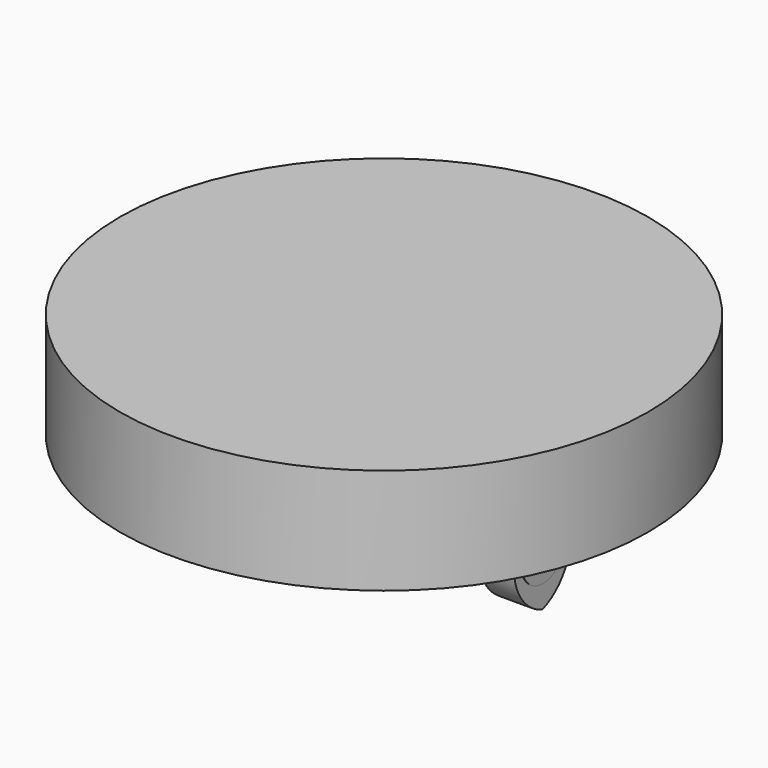
from build123d import *

# Parameters (mm, degrees)
F0_R        = 3.7479112611
F1_DEPTH    = 1.5
F3_DEPTH    = 1.5
F5_D        = 0.75
F6_T1_DEPTH = 4.2451243754
F8_R        = 0.375
F9_DEPTH    = 4.5


# Not quite as in the source:
# - a fillet or chamfer that OpenCascade refuses, or shapes differently, is made with other operations: its cross-section is extruded or revolved along the edge and cut away or added


with BuildPart() as f1:
    # F0 (on Top) → F1 (new body)
    with BuildSketch(Plane.XY):
        Circle(F0_R)
    extrude(amount=-F1_DEPTH)

    # F2 (on face) → F3 (join)
    with BuildSketch(Plane(origin=(0, 0, -1.5), x_dir=(1, 0, 0), z_dir=(0, 0, -1))):
        Polygon((-2.2448661039, -0.5004639388), (-1.7497417284, -0.5004639388), (-1.7497417284, 0), (-1.7497417284, 0.5004639388), (-2.2448661039, 0.5004639388), align=None)
    extrude(amount=F3_DEPTH)

    # F5 (through all)
    with Locations(Plane.YZ.offset(-1.7497417284)):
        with Locations((0, -2.2526816465)):
            Hole(F5_D / 2)

    # F6: fillet of radius 0.75 on 2 edges, made by hand

    # F6_s2 → F6_t1 (cut)
    with BuildSketch(Plane.YZ.offset(-4.1198661039)):
        with BuildLine():
            ThreePointArc((-0.5004639388, -2.25), (-0.2807940247, -2.7803300859), (0.2495360612, -3))
            Line((0.2495360612, -3), (-0.5004639388, -3))
            Line((-0.5004639388, -3), (-0.5004639388, -2.25))
        make_face()
        with BuildLine():
            ThreePointArc((0.5004639388, -2.25), (0.2807940247, -2.7803300859), (-0.2495360612, -3))
            Line((-0.2495360612, -3), (0.5004639388, -3))
            Line((0.5004639388, -3), (0.5004639388, -2.25))
        make_face()
    extrude(amount=F6_T1_DEPTH, mode=Mode.SUBTRACT)

    # F7: F1 across plane


with BuildPart() as f1_1:
    add(f1.part)
    add(f1.part.mirror(Plane.YZ))


with BuildPart() as f9:
    # F8 (on face) → F9 (new body)
    with BuildSketch(Plane(origin=(-2.2448661039, 0, 0), x_dir=(0, -1, 0), z_dir=(-1, 0, 0))):
        with Locations((0, -2.2526816465)):
            Circle(F8_R)
    extrude(amount=-F9_DEPTH)


solid = Compound([f1_1.part, f9.part])
